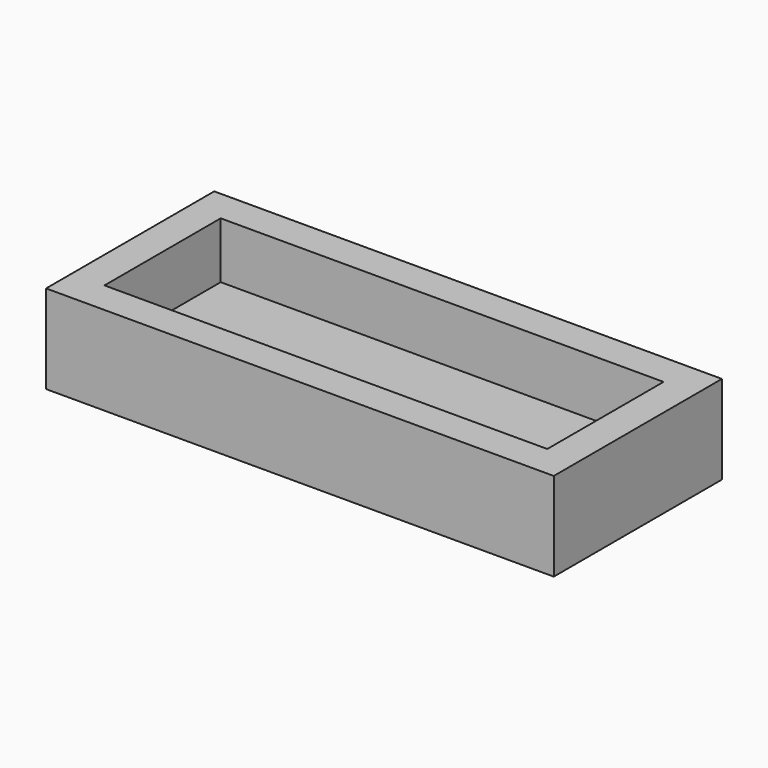
from build123d import *

# Parameters (mm, degrees)
F1_W     = 65.024
F1_H     = 21.336
F2_DEPTH = 4.7625
F1_H_2   = 4.7625
F3_DEPTH = 13.0175


# Not quite as in the source:
# - a variable given as a bare number and used for a length is read in inches; the dataset says mm whatever the document's units were


with BuildPart() as f2:
    # F1 (on Top) → F2 (new body)
    with BuildSketch(Plane.XY):
        Rectangle(F1_W, F1_H)
    extrude(amount=F2_DEPTH)

    # F1 (on Top) → F3 (join)
    with BuildSketch(Plane.XY):
        Polygon((37.2745, 15.4305), (-37.2745, 15.4305), (-37.2745, 10.668), (-32.512, 10.668), (32.512, 10.668), (37.2745, 10.668), align=None)
        Polygon((37.2745, -15.4305), (37.2745, 10.668), (32.512, 10.668), (32.512, -10.668), (32.512, -15.4305), align=None)
        with Locations((0, -13.04925)):
            Rectangle(F1_W, F1_H_2)
        Polygon((-32.512, 10.668), (-37.2745, 10.668), (-37.2745, -15.4305), (-32.512, -15.4305), (-32.512, -10.668), align=None)
    extrude(amount=F3_DEPTH)


solid = f2.part
